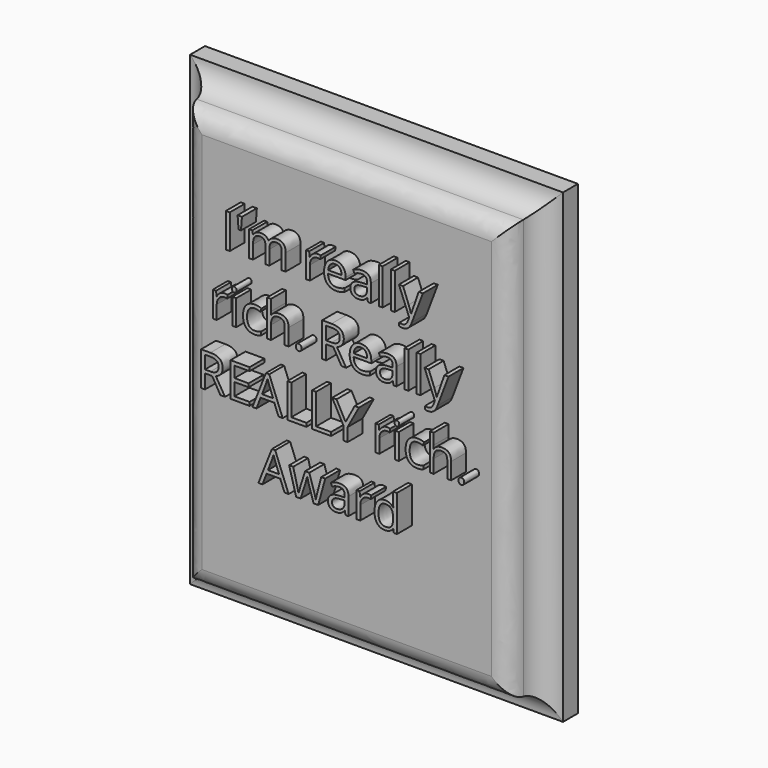
from build123d import *

# Parameters (mm, degrees)
F0_W         = 101.6
F0_H         = 127
F1_DEPTH     = 15.24
F2_W         = 101.6
F2_H         = 127
F2_W_2       = 88.9
F2_H_2       = 114.3
F3_DEPTH     = 10.16
F4_R         = 6.34999
F5_R         = 5.08
F6_TEXT_SIZE = 13.0096930488
F7_DEPTH     = 5.08


# Not quite as in the source:
# - a fillet or chamfer is up to 0.001 mm smaller than in the source, because OpenCascade refuses the exact size
# - Text() gives the source's letters only with a copy of the font that has no kerning and outlines rounded to 1/6400 em; it was checked with that copy


with BuildPart() as f1:
    # F0 (on Front) → F1 (new body)
    with BuildSketch(Plane.XZ):
        with Locations((-50.8, 63.5)):
            Rectangle(F0_W, F0_H)
    extrude(amount=F1_DEPTH)

    # F2 (on face) → F3 (cut)
    with BuildSketch(Plane.XZ.offset(15.24)):
        with Locations((-50.8, 63.5)):
            Rectangle(F2_W, F2_H)
        with Locations((-50.8, 63.5)):
            Rectangle(F2_W_2, F2_H_2, mode=Mode.SUBTRACT)
    extrude(amount=-F3_DEPTH, mode=Mode.SUBTRACT)

    # F4 (radius 6.35 in the source; OpenCascade refuses exactly that, so slightly less here)
    f4_edges = [f1.edges().sort_by_distance(p)[0] for p in [
        (-50.8, -5.08, 120.65),
        (-6.35, -5.08, 63.5),
        (-95.25, -5.08, 63.5),
        (-50.8, -5.08, 6.35),
    ]]
    fillet(f4_edges, radius=F4_R)

    # F5
    f5_edges = [f1.edges().sort_by_distance(p)[0] for p in [
        (-6.35, -15.24, 63.5),
        (-50.8, -15.24, 6.35),
        (-95.25, -15.24, 63.5),
        (-50.8, -15.24, 120.65),
    ]]
    fillet(f5_edges, radius=F5_R)

    # F6 (on face) → F7 (join)
    with BuildSketch(Plane.XZ.offset(15.24)):
        with Locations((-80.939799818, 93.5737956791)):
            Text("I'm really", F6_TEXT_SIZE, font='Open Sans', text_align=(TextAlign.LEFT, TextAlign.BOTTOM))
        with Locations((-84.3202872461, 75.8806131327)):
            Text('rich. Really', F6_TEXT_SIZE, font='Open Sans', text_align=(TextAlign.LEFT, TextAlign.BOTTOM))
        with Locations((-87.7007746743, 58.1874305863)):
            Text('REALLY rich.', F6_TEXT_SIZE, font='Open Sans', text_align=(TextAlign.LEFT, TextAlign.BOTTOM))
        with Locations((-70.7983375335, 40.4942480399)):
            Text('Award', F6_TEXT_SIZE, font='Open Sans', text_align=(TextAlign.LEFT, TextAlign.BOTTOM))
    extrude(amount=F7_DEPTH)


solid = f1.part
